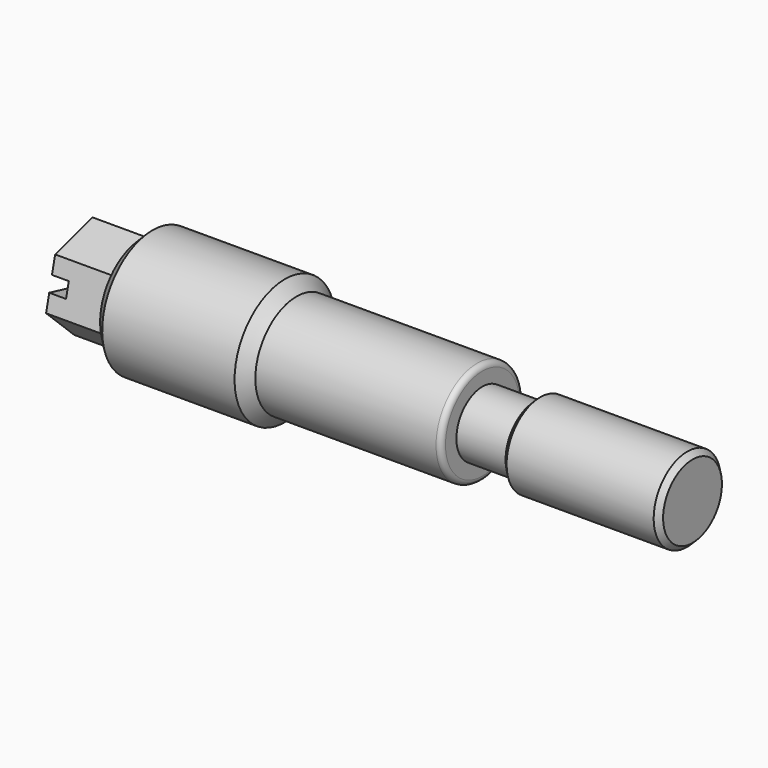
from build123d import *

# Parameters (mm, degrees)
F2_R     = 8.471957502
F3_DEPTH = 5.6
F4_SIZE  = 1.09999
F5_SIZE  = 1
F6_SIZE  = 0.5
F7_R     = 0.5
F9_DEPTH = 1.6


# Not quite as in the source:
# - a fillet or chamfer is up to 0.001 mm smaller than in the source, because OpenCascade refuses the exact size


with BuildPart() as f1:
    # F0 (on Front) → F1 (revolve)
    with BuildSketch(Plane.XZ):
        Polygon((-58, 0), (0, 0), (0, 4), (-15, 4), (-15, 3.1), (-20, 3.1), (-20, 4.9), (-37.7, 4.9), (-37.7, 6), (-52.4, 6), (-52.4, 5), (-58, 5), align=None)
    revolve(axis=Axis((-31.3887451561, 0, 0), (-1, 0, 0)))

    # F2 (on face) → F3 (cut, through all)
    with BuildSketch(Plane(origin=(-58, 0, 0), x_dir=(0, -1, 0), z_dir=(-1, 0, 0))):
        Circle(F2_R)
        Polygon((-1.0790139268, 4.4909979157), (3.34981132, 3.1799524295), (4.4288252468, -1.3110454863), (1.0790139268, -4.4909979157), (-3.34981132, -3.1799524295), (-4.4288252468, 1.3110454863), align=None, mode=Mode.SUBTRACT)
    extrude(amount=-F3_DEPTH, mode=Mode.SUBTRACT)

    # F4 (size 1.1 in the source; OpenCascade refuses exactly that, so slightly less here)
    f4_edges = [f1.edges().sort_by_distance(p)[0] for p in [
        (-37.7, 0, -6),
    ]]
    chamfer(f4_edges, length=F4_SIZE)

    # F5
    f5_edges = [f1.edges().sort_by_distance(p)[0] for p in [
        (-52.4, 0, -6),
    ]]
    chamfer(f5_edges, length=F5_SIZE)

    # F6
    f6_edges = [f1.edges().sort_by_distance(p)[0] for p in [
        (0, 0, -4),
        (-15, 0, -4),
    ]]
    chamfer(f6_edges, length=F6_SIZE)

    # F7
    f7_edges = [f1.edges().sort_by_distance(p)[0] for p in [
        (-20, 0, -4.9),
    ]]
    fillet(f7_edges, radius=F7_R)

    # F8 (on face) → F9 (cut)
    with BuildSketch(Plane(origin=(-58, 0, 0), x_dir=(0, -1, 0), z_dir=(-1, 0, 0))):
        Polygon((-4.0528476409, -0.253822772), (-3.7257889258, -1.6150841712), (4.0528476409, 0.253822772), (3.7257889258, 1.6150841712), align=None)
    extrude(amount=-F9_DEPTH, mode=Mode.SUBTRACT)


solid = f1.part
